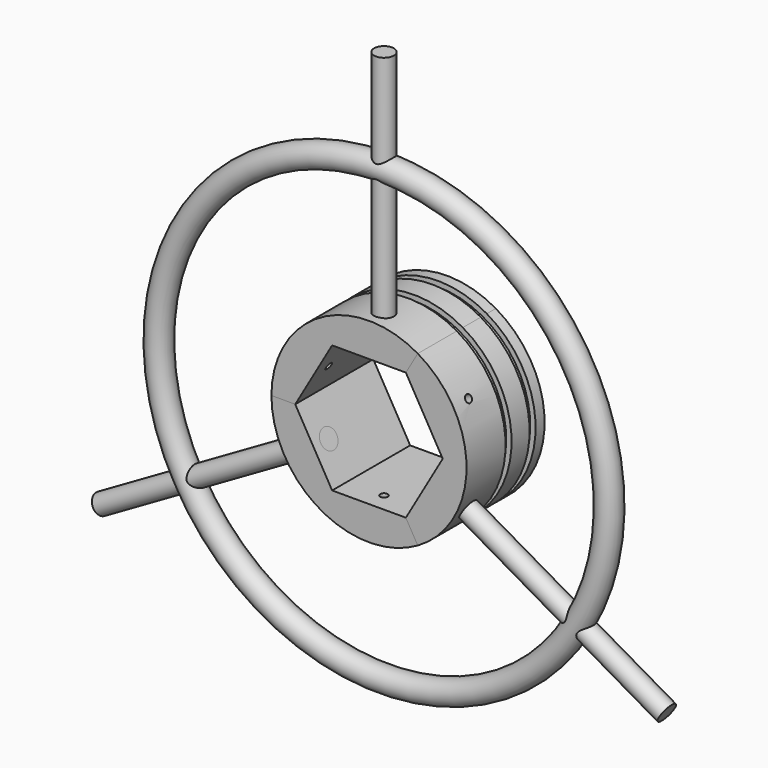
from build123d import *
from build123d import SkipClean  # not in build123d's __all__

# Parameters (mm, degrees)
F1_DEPTH = 65
F3_D     = 5
F4_R     = 6.5955625586
F5_DEPTH = 175
F6_COUNT = 3
F7_W     = 5
F7_H     = 6.1170028751
F9_R     = 8


# Not quite as in the source:
# - a feature names something its author has since deleted; it is built from what else it names


with BuildPart() as f1:
    # F0 (on Front) → F1 (new body)
    with BuildSketch(Plane.XZ):
        with BuildLine():
            Line((-49.132507908, 0), (-24.566253954, 42.55))
            Line((-24.566253954, 42.55), (24.566253954, 42.55))
            Line((24.566253954, 42.55), (32.5, 56.291651246))
            ThreePointArc((32.5, 56.291651246), (-32.5, 56.291651246), (-65, 0))
            Line((-65, 0), (-49.132507908, 0))
        make_face()
    extrude(amount=-F1_DEPTH)

    # F3 (through all)
    with Locations(Plane(origin=(-36.849380931, 0, 21.275), x_dir=(0, 1, 0), z_dir=(0.8660254038, 0, -0.5))):
        with Locations((12.5, 0)):
            Hole(F3_D / 2)

    # F6: F5, F1 ×3 about axis
    f6_axis = Axis((0, 0, 0), (0, -1, 0))


with BuildPart() as f5:
    # F4 (on face) → F5 (new body)
    with BuildSketch(Plane(origin=(0, 0, 42.55), x_dir=(1, 0, 0), z_dir=(0, 0, -1))):
        with Locations((0, -12.5)):
            Circle(F4_R)
    extrude(amount=-F5_DEPTH)


with BuildPart() as f1_1:
    add(f1.part, clean=False)


with BuildPart() as f1_2:
    add(f1_1.part, clean=False)
    with SkipClean():  # cleaning this boolean's faces spoils the solid; the shape is the same uncleaned
        for i in range(1, F6_COUNT):
            add(f5.part.rotate(f6_axis, i * 360 / F6_COUNT), clean=False)
            add(f1_1.part.rotate(f6_axis, i * 360 / F6_COUNT), clean=False)

    # F7 (on Right) → F8 (revolve, cut)
    with BuildSketch(Plane.YZ):
        with Locations((55, 64.5)):
            Rectangle(F7_W, F7_H)
        with Locations((35, 64.5)):
            Rectangle(F7_W, F7_H)
    with SkipClean():  # cleaning this boolean's faces spoils the solid; the shape is the same uncleaned
        revolve(axis=Axis((0, 65, 0), (0, -1, 0)), mode=Mode.SUBTRACT)


with BuildPart() as f5_1:
    add(f5.part, clean=False)

    # F9 (on Right) → F10 (revolve)
    with BuildSketch(Plane.YZ):
        with Locations((12.5, 150)):
            Circle(F9_R)
    revolve(axis=Axis((0, 0, 0), (0, -1, 0)))


solid = Compound([f1_2.part, f5_1.part])
